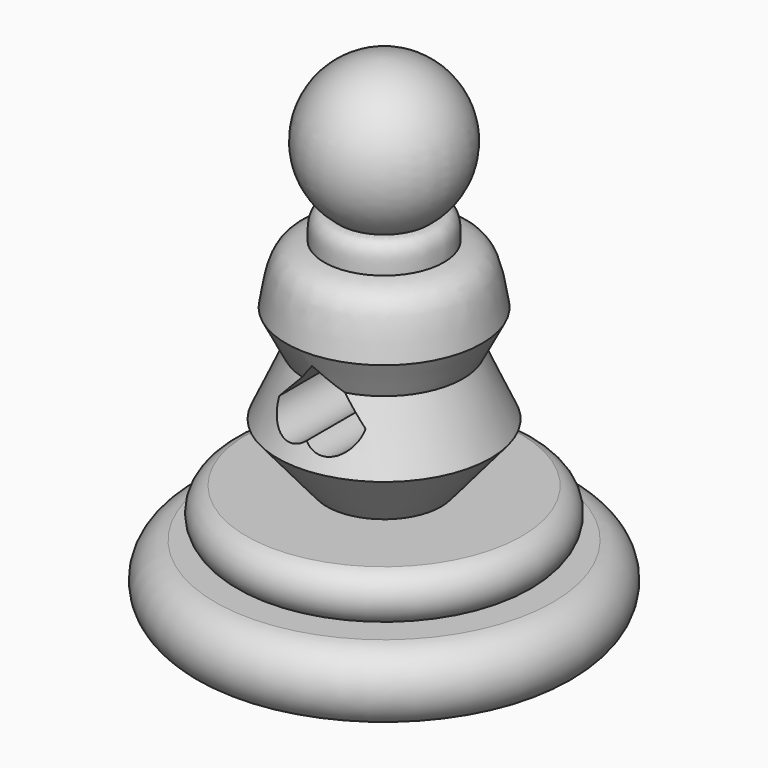
from build123d import *

# Parameters (mm, degrees)
F3_DEPTH = 31.75


# Not quite as in the source:
# - a feature names something its author has since deleted; it is built from what else it names


with BuildPart() as f1:
    # F0 (on Front) → F1 (revolve)
    with BuildSketch(Plane.XZ):
        with BuildLine():
            add(Edge.make_bspline(
                [(1.4225791464, 9.9982934775), (3.5132915341, 10.1537318423), (5.5401856361, 10.3176870642), (7.1675768375, 10.1135334914)],
                knots=[0, 0, 0, 0, 0.1307456585, 0.1307456585, 0.1307456585, 0.1307456585], degree=3))
            Line((1.4225791464, 9.9982934775), (0, 9.9982934775))
            Line((0, 9.9982934775), (0, -15.7453458756))
            Line((0, -15.7453458756), (6.844733112, -15.7453458756))
            add(Edge.make_bspline(
                [(6.844733112, -15.7453458756), (9.8138252272, -12.2815374963), (9.8018996572, -12.1859745376), (12.7709917724, -8.7221661583)],
                knots=[0, 0, 0, 0, 9.1894284399, 9.1894284399, 9.1894284399, 9.1894284399], degree=3))
            Line((12.7709917724, -8.7221661583), (9.4544900581, -1.4063537354))
            Line((9.4544900581, -1.4063537354), (11.7374207824, 3.0448461883))
            add(Edge.make_bspline(
                [(7.1675768375, 10.1135334914), (8.2006828057, 9.9839320322), (11.0535961302, 9.0746778749), (11.2645645014, 5.5467833804), (11.7374207824, 3.0448461883)],
                knots=[0.1307456585, 0.1307456585, 0.1307456585, 0.1307456585, 0.2137460581, 0.4022641918, 0.4022641918, 0.4022641918, 0.4022641918], degree=3))
        make_face()
        with BuildLine():
            Line((0, 9.9982934775), (1.4225791464, 9.9982934775))
            add(Edge.make_bspline(
                [(1.4225791464, 9.9982934775), (3.5132915341, 10.1537318423), (5.5401856361, 10.3176870642), (7.1675768375, 10.1135334914)],
                knots=[0, 0, 0, 0, 0.1307456585, 0.1307456585, 0.1307456585, 0.1307456585], degree=3))
            add(Edge.make_bspline(
                [(5.3901212251, 13.5075953739), (5.6290164894, 13.4956751346), (6.107648103, 13.4723081346), (6.7817649417, 12.9824490583), (7.1397634671, 12.0654100879), (7.1742502977, 11.0969558712), (7.177491082, 10.4812816024), (7.1675768375, 10.1135334914)],
                knots=[0, 0, 0, 0, 0.1792703508, 0.3677423577, 0.576983755, 0.7861229821, 1, 1, 1, 1], degree=3))
            Line((5.3901212251, 13.5075953739), (0, 13.5075953739))
            Line((0, 13.5075953739), (0, 11.6870473779))
            Line((0, 11.6870473779), (0, 9.9982934775))
        make_face()
        with BuildLine():
            Line((0, 13.5075953739), (5.3901212251, 13.5075953739))
            ThreePointArc((5.3901212251, 13.5075953739), (8.4224545566, 23.4216827588), (0, 29.4670473756))
            Line((0, 29.4670473756), (0, 13.5075953739))
        make_face()
    revolve(axis=Axis((0, 0, -4.1437901443), (0, 0, -1)))

    # F2 (on Front) → F3 (cut, symmetric)
    with BuildSketch(Plane.XZ):
        with BuildLine():
            ThreePointArc((-5.0167286749, -4.093704565), (-3.1493075831, -6.7330207449), (0.0495354749, -6.263281965))
            ThreePointArc((0.0495354749, -6.263281965), (3.3044071146, -6.9215070837), (5.2770635973, -4.2501635831))
            Line((5.2770635973, -4.2501635831), (0.0495354749, 1.2939639163))
            Line((0.0495354749, 1.2939639163), (-5.0167286749, -4.093704565))
        make_face()
    extrude(amount=F3_DEPTH, both=True, mode=Mode.SUBTRACT)


with BuildPart() as f5:
    # F4 (on Front) → F5 (revolve)
    with BuildSketch(Plane.XZ):
        with BuildLine():
            Line((8.57775e-05, -15.7453658836), (8.57775e-05, -29.2449350314))
            Line((8.57775e-05, -29.2449350314), (20.2102215056, -29.2449350314))
            Line((20.2102215056, -29.2449350314), (21.966146401, -29.2449350314))
            ThreePointArc((21.966146401, -29.2449350314), (23.7679662893, -24.7620009867), (20.2102215056, -21.4931013839))
            Line((20.2102215056, -21.4931013839), (16.4727318127, -21.4931013839))
            ThreePointArc((16.4727318127, -21.4931013839), (18.6177291758, -18.6192336338), (16.4727318127, -15.7453658836))
            Line((16.4727318127, -15.7453658836), (11.6290935342, -15.7453658836))
            Line((11.6290935342, -15.7453658836), (8.57775e-05, -15.7453658836))
        make_face()
    revolve(axis=Axis((8.57775e-05, 0, -26.4021651819), (0, 0, 1)))


solid = Compound([f1.part, f5.part])
